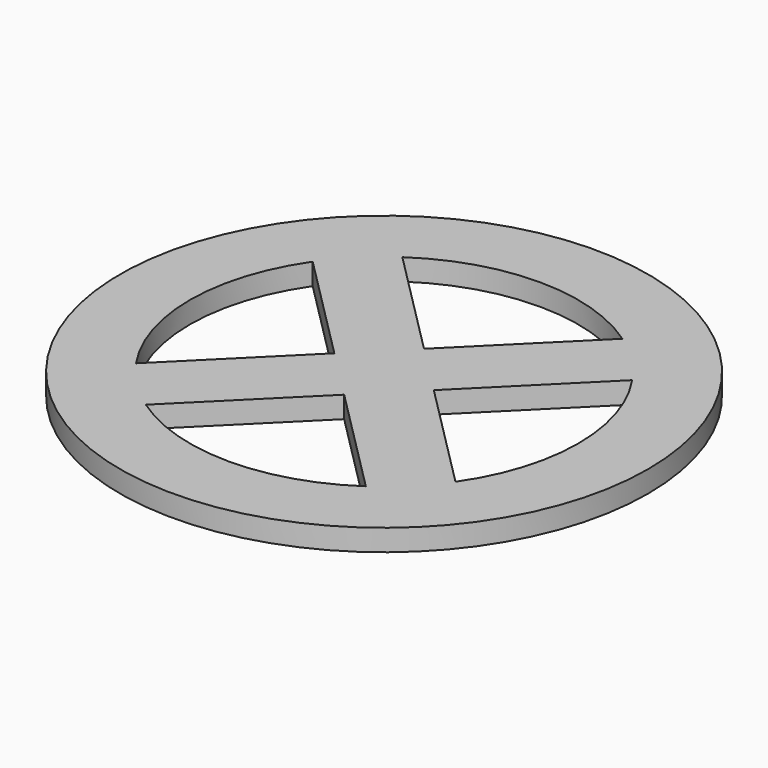
from build123d import *

# Parameters (mm, degrees)
F0_R     = 93.302436173
F1_DEPTH = 7.62


# Not quite as in the source:
# - ends of sketch curves that miss each other by under 0.0002 mm in the source are joined


with BuildPart() as f1:
    # F0 (on Top) → F1 (new body)
    with BuildSketch(Plane.XY):
        Circle(F0_R)
        with BuildLine():
            Line((-39.0521280378, -56.4777448198), (-0.032374081, -17.6012715653))
            Line((-0.032374081, -17.6012715653), (38.8440970553, -56.6210251423))
            ThreePointArc((38.8440970553, -56.6210251423), (-0.1262993869, -68.6643168805), (-39.0521280378, -56.4777448198))
        make_face(mode=Mode.SUBTRACT)
        with BuildLine():
            Line((56.477744538, -39.0521284453), (17.6012712801, -0.0323744851))
            Line((17.6012712801, -0.0323744851), (56.6210244822, 38.8440980175))
            ThreePointArc((56.6210244822, 38.8440980175), (68.6643168811, -0.1262990512), (56.477744538, -39.0521284453))
        make_face(mode=Mode.SUBTRACT)
        with BuildLine():
            ThreePointArc((-56.6210254, -38.8440966797), (-68.6643168783, 0.1263005725), (-56.4777437302, 39.0521296136))
            Line((-56.4777437302, 39.0521296136), (-17.6012714166, 0.0323766012))
            Line((-17.6012714166, 0.0323766012), (-56.6210254, -38.8440966797))
        make_face(mode=Mode.SUBTRACT)
        with BuildLine():
            Line((39.0521279012, 56.4777449142), (0.0323739658, 17.601271681))
            Line((0.0323739658, 17.601271681), (-38.8440980887, 56.6210244334))
            ThreePointArc((-38.8440980887, 56.6210244334), (0.1262986773, 68.6643168818), (39.0521279012, 56.4777449142))
        make_face(mode=Mode.SUBTRACT)
    extrude(amount=F1_DEPTH)


solid = f1.part
